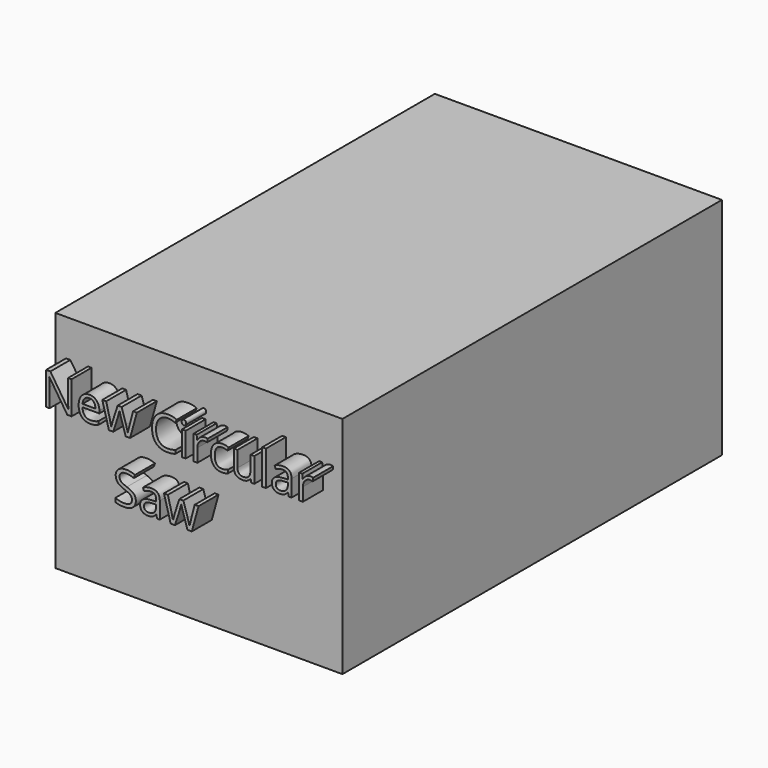
from build123d import *

# Parameters (mm, degrees)
F0_W         = 292.1
F0_H         = 228.6
F1_DEPTH     = 482.6
F2_TEXT_SIZE = 46.5460603379
F3_DEPTH     = 25.4


# Not quite as in the source:
# - Text() gives the source's letters only with a copy of the font that has no kerning and outlines rounded to 1/6400 em; it was checked with that copy


with BuildPart() as f1:
    # F0 (on Front) → F1 (new body)
    with BuildSketch(Plane.XZ):
        Rectangle(F0_W, F0_H)
    extrude(amount=F1_DEPTH)

    # F2 (on face) → F3 (join)
    with BuildSketch(Plane.XZ.offset(482.6)):
        with Locations((-139.7, 43.9074032504)):
            Text('New Circular', F2_TEXT_SIZE, font='Open Sans', text_align=(TextAlign.LEFT, TextAlign.BOTTOM))
        with Locations((-67.1317828045, -19.3952388091)):
            Text('Saw', F2_TEXT_SIZE, font='Open Sans', text_align=(TextAlign.LEFT, TextAlign.BOTTOM))
    extrude(amount=F3_DEPTH)


solid = f1.part
